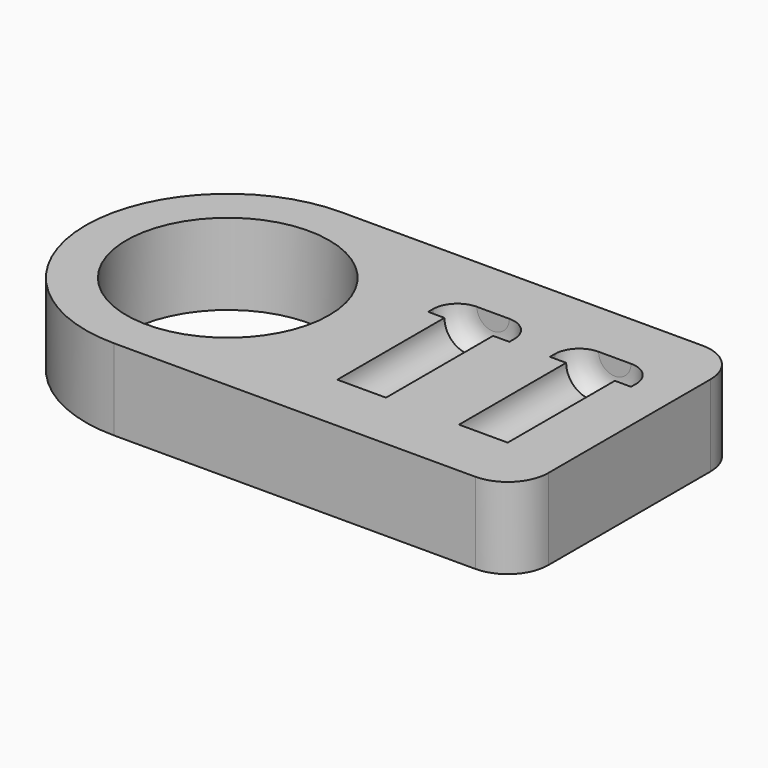
from build123d import *

# Parameters (mm, degrees)
F0_R         = 12.5
F1_DEPTH     = 10
F5_TEXT_SIZE = 5.5555555556
F6_DEPTH     = 1


# Not quite as in the source:
# - Text() gives the source's letters only with a copy of the font that has no kerning and outlines rounded to 1/6400 em; it was checked with that copy


with BuildPart() as f1:
    # F0 (on Top) → F1 (new body)
    with BuildSketch(Plane.XY):
        with BuildLine():
            ThreePointArc((0, 17.5), (5.1256313292, 5.1256313292), (17.5, 0))
            Line((17.5, 0), (62, 0))
            ThreePointArc((62, 0), (65.5355339059, 1.4644660941), (67, 5))
            Line((67, 5), (67, 30))
            ThreePointArc((67, 30), (65.5355339059, 33.5355339059), (62, 35))
            Line((62, 35), (17.5, 35))
            ThreePointArc((17.5, 35), (5.1256313292, 29.8743686708), (0, 17.5))
        make_face()
        with Locations((17.5, 17.5)):
            Circle(F0_R, mode=Mode.SUBTRACT)
    extrude(amount=F1_DEPTH)

    # F2 (on face) → F3 (revolve, cut)
    with BuildSketch(Plane.XY.offset(10)):
        with BuildLine():
            Line((42, 24), (42, 7.5))
            Line((42, 7.5), (45, 7.5))
            Line((45, 7.5), (45, 24))
            Line((45, 24), (47, 24))
            Line((47, 24), (47, 24.75))
            ThreePointArc((47, 24.75), (46.1213203436, 26.8713203436), (44, 27.75))
            Line((44, 27.75), (42, 27.75))
            Line((42, 27.75), (42, 24))
        make_face()
    revolve(axis=Axis((42, 15.75, 10), (0, 1, 0)), mode=Mode.SUBTRACT)

    # F2 (on face) → F4 (revolve, cut)
    with BuildSketch(Plane.XY.offset(10)):
        with BuildLine():
            Line((57, 24), (57, 7.5))
            Line((57, 7.5), (60, 7.5))
            Line((60, 7.5), (60, 24))
            Line((60, 24), (62, 24))
            Line((62, 24), (62, 24.75))
            ThreePointArc((62, 24.75), (61.1213203436, 26.8713203436), (59, 27.75))
            Line((59, 27.75), (57, 27.75))
            Line((57, 27.75), (57, 24))
        make_face()
    revolve(axis=Axis((57, 15.75, 10), (0, 1, 0)), mode=Mode.SUBTRACT)

    # F5 (on face) → F6 (cut)
    with BuildSketch(Plane(origin=(0, 0, 0), x_dir=(1, 0, 0), z_dir=(0, 0, -1))):
        with Locations((30, -9)):
            Text('789', F5_TEXT_SIZE, font='Open Sans', text_align=(TextAlign.LEFT, TextAlign.BOTTOM))
    extrude(amount=-F6_DEPTH, mode=Mode.SUBTRACT)


solid = f1.part
